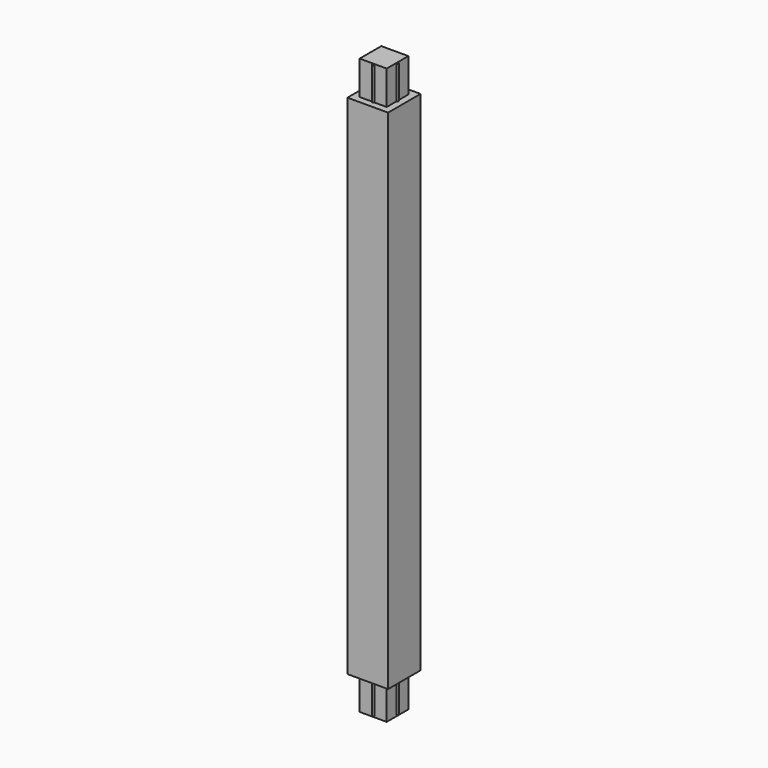
from build123d import *

# Parameters (mm, degrees)
F0_W     = 12
F0_H     = 12
F1_DEPTH = 75
F3_DEPTH = 10
F4_SIZE  = 0.3


# Not quite as in the source:
# - a pattern or mirror of a feature is missing from the dataset's text; its kind, count and spacing are read off the source's solid


with BuildPart() as f1:
    # F0 (on Top) → F1 (new body, symmetric)
    with BuildSketch(Plane.XY):
        Rectangle(F0_W, F0_H)
    extrude(amount=F1_DEPTH, both=True)

    # F2 (on face) → F3 (join)
    with BuildSketch(Plane.XY.offset(75)):
        Polygon((-0.3250005729, 4), (-4, 4), (-4, 0.325), (-4, -0.325), (-4, -4), (-0.3250005729, -4), (0.3250005729, -4), (4, -4), (4, -0.325), (4, 0.325), (4, 4), (0.3250005729, 4), align=None)
        with BuildLine():
            ThreePointArc((0.3250005729, 4), (0, 4.3250005729), (-0.3250005729, 4))
            Line((-0.3250005729, 4), (0.3250005729, 4))
        make_face()
        with BuildLine():
            Line((-4, -0.325), (-4, 0.325))
            ThreePointArc((-4, 0.325), (-4.325, 0), (-4, -0.325))
        make_face()
        with BuildLine():
            ThreePointArc((4, -0.325), (4.325, 0), (4, 0.325))
            Line((4, 0.325), (4, -0.325))
        make_face()
        with BuildLine():
            Line((0.3250005729, -4), (-0.3250005729, -4))
            ThreePointArc((-0.3250005729, -4), (0, -4.3250005729), (0.3250005729, -4))
        make_face()
    f3 = extrude(amount=F3_DEPTH)

    # F3_copies: F3 across plane
    add(f3.mirror(Plane(origin=(0, 0, 0), x_dir=(-1, 0, 0), z_dir=(0, 0, -1))))

    # F4
    f4_edges = [f1.edges().sort_by_distance(p)[0] for p in [
        (0, -4.325001, 85),
        (4.325, 0, 85),
        (0, 4.325001, 85),
        (-4.325, 0, 85),
        (-4.325, 0, -85),
        (0, -4.325001, -85),
        (4.325, 0, -85),
        (0, 4.325001, -85),
    ]]
    chamfer(f4_edges, length=F4_SIZE)


solid = f1.part
